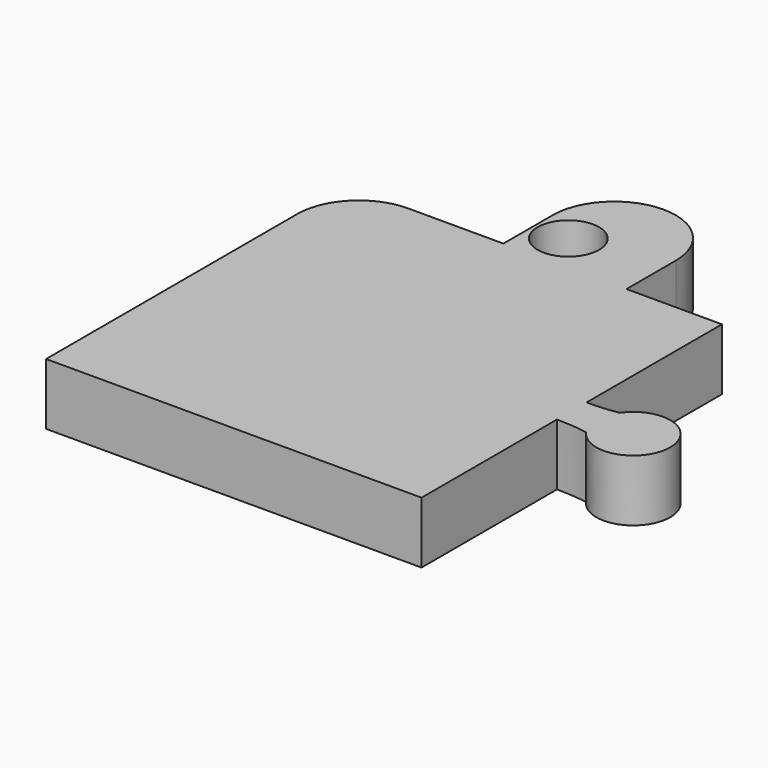
from build123d import *

# Parameters (mm, degrees)
F1_DEPTH = 5
F2_R     = 5
F3_W     = 5
F3_H     = 5
F4_DEPTH = 10
F5_R     = 4.99999
F6_R     = 2.5
F7_DEPTH = 25


# Not quite as in the source:
# - a fillet or chamfer is up to 0.001 mm smaller than in the source, because OpenCascade refuses the exact size


with BuildPart() as f1:
    # F0 (on Top) → F1 (new body)
    with BuildSketch(Plane.XY):
        with BuildLine():
            Line((2.2222189992, 32.4371969399), (2.2222189992, 33.9371969399))
            Line((2.2222189992, 33.9371969399), (2.2222189992, 35.4371969399))
            add(Edge.make_bspline(
                [(2.2222189992, 35.4371969399), (-2.7777810008, 35.4371969399), (-2.7777810008, 33.9371969399), (-2.7777810008, 32.4371969399), (2.2222189992, 32.4371969399)],
                knots=[1.5707963268, 1.5707963268, 1.5707963268, 3.1415926536, 3.1415926536, 4.7123889804, 4.7123889804, 4.7123889804], degree=2, weights=[1, 0.7071067812, 1, 0.7071067812, 1]))
        make_face()
        with BuildLine():
            add(Edge.make_bspline(
                [(2.2222189992, 32.4371969399), (3.5823095151, 32.4371969399), (4.7549905191, 32.6438848513)],
                knots=[4.7123889804, 4.7123889804, 4.7123889804, 5.2435726948, 5.2435726948, 5.2435726948], degree=2, weights=[1, 0.964937319, 1]))
            Line((2.2222189992, 32.4371969399), (2.2222189992, 30.9371969399))
            Line((2.2222189992, 30.9371969399), (4.2222189992, 30.9371969399))
            add(Edge.make_bspline(
                [(4.7549905191, 32.6438848513), (4.2222189992, 31.8736977196), (4.2222189992, 30.9371969399)],
                knots=[0.9656335287, 0.9656335287, 0.9656335287, 1.5707963268, 1.5707963268, 1.5707963268], degree=2, weights=[1, 0.9545704514, 1]))
        make_face()
        with BuildLine():
            Line((2.2222189992, 30.9371969399), (2.2222189992, 32.4371969399))
            add(Edge.make_bspline(
                [(2.2222189992, 35.4371969399), (-2.7777810008, 35.4371969399), (-2.7777810008, 33.9371969399), (-2.7777810008, 32.4371969399), (2.2222189992, 32.4371969399)],
                knots=[1.5707963268, 1.5707963268, 1.5707963268, 3.1415926536, 3.1415926536, 4.7123889804, 4.7123889804, 4.7123889804], degree=2, weights=[1, 0.7071067812, 1, 0.7071067812, 1]))
            Line((2.2222189992, 35.4371969399), (2.2222189992, 46.1871969399))
            Line((2.2222189992, 46.1871969399), (-28.2777810008, 46.1871969399))
            Line((-28.2777810008, 46.1871969399), (-28.2777810008, 15.6871969399))
            Line((-28.2777810008, 15.6871969399), (2.2222189992, 15.6871969399))
            Line((2.2222189992, 15.6871969399), (2.2222189992, 26.4371969399))
            add(Edge.make_bspline(
                [(2.2222189992, 29.4371969399), (-2.7777810008, 29.4371969399), (-2.7777810008, 27.9371969399), (-2.7777810008, 26.4371969399), (2.2222189992, 26.4371969399)],
                knots=[4.7123889804, 4.7123889804, 4.7123889804, 6.2831853072, 6.2831853072, 7.853981634, 7.853981634, 7.853981634], degree=2, weights=[1, 0.7071067812, 1, 0.7071067812, 1]))
            Line((2.2222189992, 29.4371969399), (2.2222189992, 30.9371969399))
        make_face()
        with BuildLine():
            Line((4.2222189992, 30.9371969399), (2.2222189992, 30.9371969399))
            Line((2.2222189992, 30.9371969399), (2.2222189992, 29.4371969399))
            add(Edge.make_bspline(
                [(4.7549905191, 29.2305090285), (3.5823095151, 29.4371969399), (2.2222189992, 29.4371969399)],
                knots=[4.181205266, 4.181205266, 4.181205266, 4.7123889804, 4.7123889804, 4.7123889804], degree=2, weights=[1, 0.964937319, 1]))
            add(Edge.make_bspline(
                [(4.2222189992, 30.9371969399), (4.2222189992, 30.0006961603), (4.7549905191, 29.2305090285)],
                knots=[1.5707963268, 1.5707963268, 1.5707963268, 2.1759591249, 2.1759591249, 2.1759591249], degree=2, weights=[1, 0.9545704514, 1]))
        make_face()
        with BuildLine():
            add(Edge.make_bspline(
                [(7.2222189992, 33.9371969399), (5.6496300407, 33.9371969399), (4.7549905191, 32.6438848513)],
                knots=[0, 0, 0, 0.9656335287, 0.9656335287, 0.9656335287], degree=2, weights=[1, 0.8856906826, 1]))
            add(Edge.make_bspline(
                [(4.7549905191, 32.6438848513), (7.2222189992, 33.0787399396), (7.2222189992, 33.9371969399)],
                knots=[5.2435726948, 5.2435726948, 5.2435726948, 6.2831853072, 6.2831853072, 6.2831853072], degree=2, weights=[1, 0.867915406, 1]))
        make_face()
        with BuildLine():
            add(Edge.make_bspline(
                [(4.7549905191, 32.6438848513), (7.2222189992, 33.0787399396), (7.2222189992, 33.9371969399)],
                knots=[5.2435726948, 5.2435726948, 5.2435726948, 6.2831853072, 6.2831853072, 6.2831853072], degree=2, weights=[1, 0.867915406, 1]))
            add(Edge.make_bspline(
                [(4.7549905191, 32.6438848513), (4.2222189992, 31.8736977196), (4.2222189992, 30.9371969399)],
                knots=[0.9656335287, 0.9656335287, 0.9656335287, 1.5707963268, 1.5707963268, 1.5707963268], degree=2, weights=[1, 0.9545704514, 1]))
            Line((4.2222189992, 30.9371969399), (7.2222189992, 30.9371969399))
            Line((7.2222189992, 30.9371969399), (7.2222189992, 33.9371969399))
        make_face()
        with BuildLine():
            add(Edge.make_bspline(
                [(7.2222189992, 27.9371969399), (10.2222189992, 27.9371969399), (10.2222189992, 30.9371969399), (10.2222189992, 33.9371969399), (7.2222189992, 33.9371969399)],
                knots=[3.1415926536, 3.1415926536, 3.1415926536, 4.7123889804, 4.7123889804, 6.2831853072, 6.2831853072, 6.2831853072], degree=2, weights=[1, 0.7071067812, 1, 0.7071067812, 1]))
            Line((7.2222189992, 33.9371969399), (7.2222189992, 30.9371969399))
            Line((7.2222189992, 30.9371969399), (7.2222189992, 27.9371969399))
        make_face()
        with BuildLine():
            Line((2.2222189992, 27.9371969399), (2.2222189992, 29.4371969399))
            add(Edge.make_bspline(
                [(2.2222189992, 29.4371969399), (-2.7777810008, 29.4371969399), (-2.7777810008, 27.9371969399), (-2.7777810008, 26.4371969399), (2.2222189992, 26.4371969399)],
                knots=[4.7123889804, 4.7123889804, 4.7123889804, 6.2831853072, 6.2831853072, 7.853981634, 7.853981634, 7.853981634], degree=2, weights=[1, 0.7071067812, 1, 0.7071067812, 1]))
            Line((2.2222189992, 26.4371969399), (2.2222189992, 27.9371969399))
        make_face()
        with BuildLine():
            Line((7.2222189992, 30.9371969399), (4.2222189992, 30.9371969399))
            add(Edge.make_bspline(
                [(4.2222189992, 30.9371969399), (4.2222189992, 30.0006961603), (4.7549905191, 29.2305090285)],
                knots=[1.5707963268, 1.5707963268, 1.5707963268, 2.1759591249, 2.1759591249, 2.1759591249], degree=2, weights=[1, 0.9545704514, 1]))
            add(Edge.make_bspline(
                [(7.2222189992, 27.9371969399), (7.2222189992, 28.7956539402), (4.7549905191, 29.2305090285)],
                knots=[3.1415926536, 3.1415926536, 3.1415926536, 4.181205266, 4.181205266, 4.181205266], degree=2, weights=[1, 0.867915406, 1]))
            Line((7.2222189992, 27.9371969399), (7.2222189992, 30.9371969399))
        make_face()
        with BuildLine():
            add(Edge.make_bspline(
                [(4.7549905191, 29.2305090285), (5.6496300407, 27.9371969399), (7.2222189992, 27.9371969399)],
                knots=[2.1759591249, 2.1759591249, 2.1759591249, 3.1415926536, 3.1415926536, 3.1415926536], degree=2, weights=[1, 0.8856906826, 1]))
            add(Edge.make_bspline(
                [(7.2222189992, 27.9371969399), (7.2222189992, 28.7956539402), (4.7549905191, 29.2305090285)],
                knots=[3.1415926536, 3.1415926536, 3.1415926536, 4.181205266, 4.181205266, 4.181205266], degree=2, weights=[1, 0.867915406, 1]))
        make_face()
    extrude(amount=F1_DEPTH)

    # F2
    f2_edges = [f1.edges().sort_by_distance(p)[0] for p in [
        (-28.277781, 46.187197, 2.5),
    ]]
    fillet(f2_edges, radius=F2_R)

    # F3 (on face) → F4 (join)
    with BuildSketch(Plane(origin=(0, 46.1871969399, 0), x_dir=(-1, 0, 0), z_dir=(0, 1, 0))):
        with Locations((13.0277810008, 2.5)):
            Rectangle(F3_W, F3_H)
        with Locations((8.0277810008, 2.5)):
            Rectangle(F3_W, F3_H)
    extrude(amount=F4_DEPTH)

    # F5 (radius 5 in the source; OpenCascade refuses exactly that, so slightly less here)
    f5_edges = [f1.edges().sort_by_distance(p)[0] for p in [
        (-15.527781, 56.187197, 2.5),
        (-5.527781, 56.187197, 2.5),
    ]]
    fillet(f5_edges, radius=F5_R)

    # F6 (on face) → F7 (cut)
    with BuildSketch(Plane.XY.offset(5)):
        with Locations((-12.7509618178, 49.3081174791)):
            Circle(F6_R)
    extrude(amount=-F7_DEPTH, mode=Mode.SUBTRACT)


solid = f1.part
